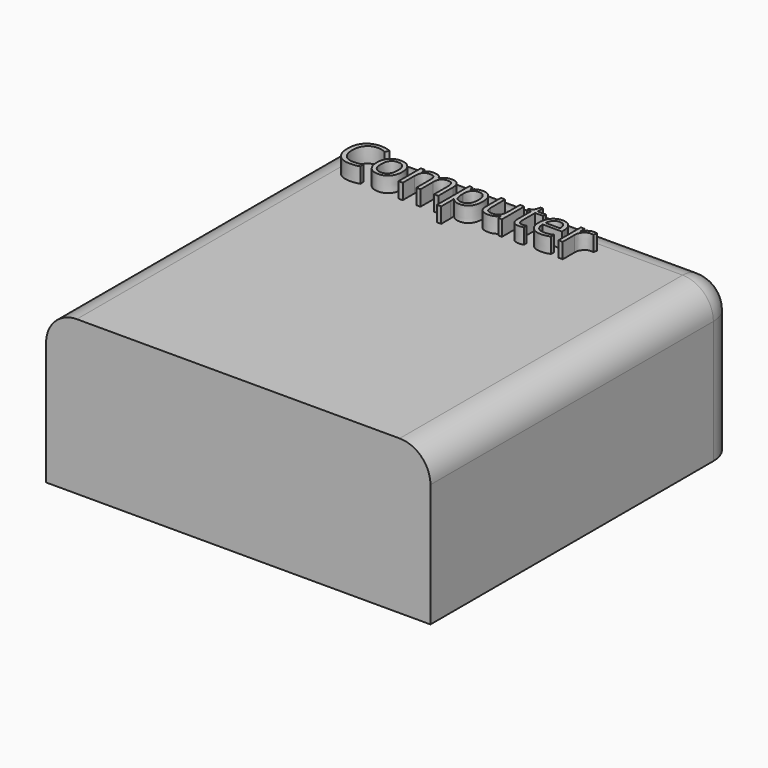
from build123d import *

# Parameters (mm, degrees)
F0_W         = 63.5
F0_H         = 63.5
F1_DEPTH     = 25.4
F2_R         = 5.08
F3_TEXT_SIZE = 8.6067757369
F4_DEPTH     = 2.54


# Not quite as in the source:
# - Text() gives the source's letters only with a copy of the font that has no kerning and outlines rounded to 1/6400 em; it was checked with that copy


with BuildPart() as f1:
    # F0 (on Top) → F1 (new body)
    with BuildSketch(Plane.XY):
        Rectangle(F0_W, F0_H)
    extrude(amount=F1_DEPTH)

    # F2
    f2_edges = [f1.edges().sort_by_distance(p)[0] for p in [
        (-31.75, 31.75, 12.7),
        (31.75, 31.75, 12.7),
        (0, 31.75, 25.4),
        (-31.75, 0, 25.4),
        (31.75, 0, 25.4),
    ]]
    fillet(f2_edges, radius=F2_R)

    # F3 (on face) → F4 (join)
    with BuildSketch(Plane.XY.offset(25.4)):
        with Locations((-26.67, 20.4731214694)):
            Text('Computer', F3_TEXT_SIZE, font='Open Sans', text_align=(TextAlign.LEFT, TextAlign.BOTTOM))
    extrude(amount=F4_DEPTH)


solid = f1.part
